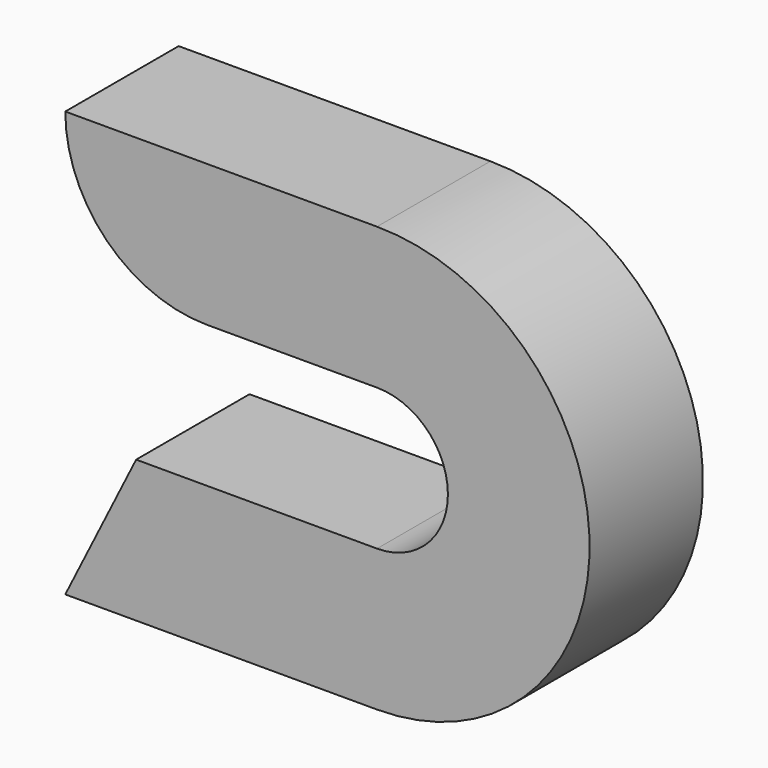
from build123d import *

# Parameters (mm, degrees)
F0_W     = 15.24
F0_H     = 12.7
F1_DEPTH = 6.35


# Not quite as in the source:
# - a feature names something its author has since deleted; it is built from what else it names


with BuildPart() as f1:
    # F0 (on Front) → F1 (new body, symmetric)
    with BuildSketch(Plane.XZ):
        Polygon((-11.5497628391, 12.7), (-17.8997628391, 0), (10.0402371609, 0), (10.0402371609, 12.7), align=None)
        with BuildLine():
            Line((10.0402371609, 12.7), (10.0402371609, 0))
            ThreePointArc((10.0402371609, 0), (29.0902371609, 19.05), (10.0402371609, 38.1))
            Line((10.0402371609, 38.1), (10.0402371609, 25.4))
            ThreePointArc((10.0402371609, 25.4), (16.3902371609, 19.05), (10.0402371609, 12.7))
        make_face()
        with Locations((2.4202371609, 31.75)):
            Rectangle(F0_W, F0_H)
        with BuildLine():
            Line((-5.1997628391, 25.4), (-5.1997628391, 38.1))
            Line((-5.1997628391, 38.1), (-17.8997628391, 38.1))
            ThreePointArc((-17.8997628391, 38.1), (-14.1800189601, 29.1197438789), (-5.1997628391, 25.4))
        make_face()
    extrude(amount=F1_DEPTH, both=True)


solid = f1.part
